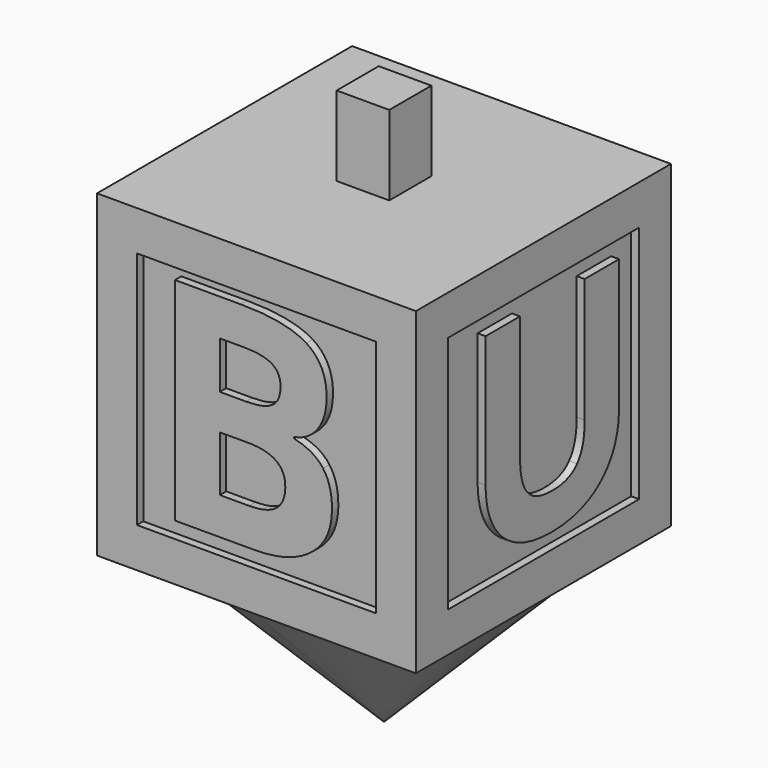
from build123d import *

# Parameters (mm, degrees)
F0_W      = 50.8
F0_H      = 50.8
F1_DEPTH  = 50.8
F2_W      = 38.1
F2_H      = 38.1
F3_DEPTH  = 1.27
F4_W      = 38.1
F4_H      = 38.1
F5_DEPTH  = 1.27
F6_W      = 38.1
F6_H      = 38.1
F7_DEPTH  = 1.27
F8_W      = 38.1
F8_H      = 38.1
F9_DEPTH  = 1.27
F10_W     = 8.382
F10_H     = 8.382
F11_DEPTH = 12.7
F13_DEPTH = 25.4
F14_SIZE  = 25.39999


# Not quite as in the source:
# - a fillet or chamfer is up to 0.001 mm smaller than in the source, because OpenCascade refuses the exact size


with BuildPart() as f1:
    # F0 (on Top) → F1 (new body)
    with BuildSketch(Plane.XY):
        Rectangle(F0_W, F0_H)
    extrude(amount=F1_DEPTH)

    # F2 (on face) → F3 (cut)
    with BuildSketch(Plane.XZ.offset(25.4)):
        with Locations((0, 25.4)):
            Rectangle(F2_W, F2_H)
        with BuildLine():
            Line((-12.9850329568, 8.9432131499), (-12.9850329568, 42.6816119349))
            Line((-12.9850329568, 42.6816119349), (-2.484703985, 42.6816119349))
            add(Edge.make_bspline(
                [(-2.484703985, 42.6816119349), (4.6927360717, 42.6816119349), (7.9343988133, 40.6398813015)],
                knots=[0, 0, 0, 1, 1, 1], degree=2))
            add(Edge.make_bspline(
                [(7.9343988133, 40.6398813015), (11.176061555, 38.5981506681), (11.176061555, 34.1454795218)],
                knots=[0, 0, 0, 1, 1, 1], degree=2))
            add(Edge.make_bspline(
                [(11.176061555, 34.1454795218), (11.176061555, 31.1179585102), (9.7582956179, 29.1796066431)],
                knots=[0, 0, 0, 1, 1, 1], degree=2))
            add(Edge.make_bspline(
                [(9.7582956179, 29.1796066431), (8.3405296807, 27.2412547759), (5.9849706498, 26.8498923037)],
                knots=[0, 0, 0, 1, 1, 1], degree=2))
            Line((5.9849706498, 26.8498923037), (5.9849706498, 26.6209821784))
            add(Edge.make_bspline(
                [(5.9849706498, 26.6209821784), (9.1897124035, 25.9047150123), (10.6111704394, 23.9442105523)],
                knots=[0, 0, 0, 1, 1, 1], degree=2))
            add(Edge.make_bspline(
                [(10.6111704394, 23.9442105523), (12.0326284753, 21.9837060924), (12.0326284753, 18.7272749556)],
                knots=[0, 0, 0, 1, 1, 1], degree=2))
            add(Edge.make_bspline(
                [(12.0326284753, 18.7272749556), (12.0326284753, 14.1121514623), (8.694971165, 11.5276823061)],
                knots=[0, 0, 0, 1, 1, 1], degree=2))
            add(Edge.make_bspline(
                [(8.694971165, 11.5276823061), (5.3573138547, 8.9432131499), (-0.3654392769, 8.9432131499)],
                knots=[0, 0, 0, 1, 1, 1], degree=2))
            Line((-0.3654392769, 8.9432131499), (-12.9850329568, 8.9432131499))
        make_face(mode=Mode.SUBTRACT)
        with BuildLine():
            Line((-5.8297454929, 36.8185590491), (-5.8297454929, 29.3162142985))
            Line((-5.8297454929, 29.3162142985), (-1.6798264478, 29.3162142985))
            add(Edge.make_bspline(
                [(-1.6798264478, 29.3162142985), (1.2295474023, 29.3162142985), (2.5328582768, 30.2170864044)],
                knots=[0, 0, 0, 1, 1, 1], degree=2))
            add(Edge.make_bspline(
                [(2.5328582768, 30.2170864044), (3.8361691513, 31.1179585102), (3.8361691513, 33.1929180328)],
                knots=[0, 0, 0, 1, 1, 1], degree=2))
            add(Edge.make_bspline(
                [(3.8361691513, 33.1929180328), (3.8361691513, 35.1349619988), (2.4184032142, 35.9767605239)],
                knots=[0, 0, 0, 1, 1, 1], degree=2))
            add(Edge.make_bspline(
                [(2.4184032142, 35.9767605239), (1.0006372771, 36.8185590491), (-2.07118892, 36.8185590491)],
                knots=[0, 0, 0, 1, 1, 1], degree=2))
            Line((-2.07118892, 36.8185590491), (-5.8297454929, 36.8185590491))
        make_face()
        with BuildLine():
            Line((-1.3992269394, 23.64515055), (-5.8297454929, 23.64515055))
            Line((-5.8297454929, 23.64515055), (-5.8297454929, 14.8505712213))
            Line((-5.8297454929, 14.8505712213), (-1.1703168141, 14.8505712213))
            add(Edge.make_bspline(
                [(-1.1703168141, 14.8505712213), (1.7833622215, 14.8505712213), (3.1900518623, 15.9803534524)],
                knots=[0, 0, 0, 1, 1, 1], degree=2))
            add(Edge.make_bspline(
                [(3.1900518623, 15.9803534524), (4.596741503, 17.1101356836), (4.596741503, 19.4435421217)],
                knots=[0, 0, 0, 1, 1, 1], degree=2))
            add(Edge.make_bspline(
                [(4.596741503, 19.4435421217), (4.596741503, 23.64515055), (-1.3992269394, 23.64515055)],
                knots=[0, 0, 0, 1, 1, 1], degree=2))
        make_face()
    extrude(amount=-F3_DEPTH, mode=Mode.SUBTRACT)

    # F4 (on face) → F5 (cut)
    with BuildSketch(Plane.YZ.offset(25.4)):
        with Locations((0, 25.4)):
            Rectangle(F4_W, F4_H)
        with BuildLine():
            Line((8.2110515278, 41.6381866004), (15.0563287647, 41.6381866004))
            Line((15.0563287647, 41.6381866004), (15.0563287647, 20.6913548071))
            add(Edge.make_bspline(
                [(15.0563287647, 20.6913548071), (15.0563287647, 17.098647189), (13.4513025803, 14.3988018192)],
                knots=[0, 0, 0, 1, 1, 1], degree=2))
            add(Edge.make_bspline(
                [(13.4513025803, 14.3988018192), (11.8462763959, 11.6989564493), (8.8098361308, 10.2569130563)],
                knots=[0, 0, 0, 1, 1, 1], degree=2))
            add(Edge.make_bspline(
                [(8.8098361308, 10.2569130563), (5.7733958658, 8.8148696632), (1.6350502071, 8.8148696632)],
                knots=[0, 0, 0, 1, 1, 1], degree=2))
            add(Edge.make_bspline(
                [(1.6350502071, 8.8148696632), (-4.6078993227, 8.8148696632), (-8.0624258786, 12.0178358237)],
                knots=[0, 0, 0, 1, 1, 1], degree=2))
            add(Edge.make_bspline(
                [(-8.0624258786, 12.0178358237), (-11.5169524345, 15.2208019843), (-11.5169524345, 20.776389307)],
                knots=[0, 0, 0, 1, 1, 1], degree=2))
            Line((-11.5169524345, 20.776389307), (-11.5169524345, 41.6381866004))
            Line((-11.5169524345, 41.6381866004), (-4.6787614059, 41.6381866004))
            Line((-4.6787614059, 41.6381866004), (-4.6787614059, 21.81806193))
            add(Edge.make_bspline(
                [(-4.6787614059, 21.81806193), (-4.6787614059, 18.0765439371), (-3.1729421379, 16.3262504822)],
                knots=[0, 0, 0, 1, 1, 1], degree=2))
            add(Edge.make_bspline(
                [(-3.1729421379, 16.3262504822), (-1.66712287, 14.5759570272), (1.8122054151, 14.5759570272)],
                knots=[0, 0, 0, 1, 1, 1], degree=2))
            add(Edge.make_bspline(
                [(1.8122054151, 14.5759570272), (5.178154367, 14.5759570272), (6.6946029474, 16.3368797946)],
                knots=[0, 0, 0, 1, 1, 1], degree=2))
            add(Edge.make_bspline(
                [(6.6946029474, 16.3368797946), (8.2110515278, 18.0978025621), (8.2110515278, 21.8605791799)],
                knots=[0, 0, 0, 1, 1, 1], degree=2))
            Line((8.2110515278, 21.8605791799), (8.2110515278, 41.6381866004))
        make_face(mode=Mode.SUBTRACT)
    extrude(amount=-F5_DEPTH, mode=Mode.SUBTRACT)

    # F6 (on face) → F7 (cut)
    with BuildSketch(Plane(origin=(0, 25.4, 0), x_dir=(-1, 0, 0), z_dir=(0, 1, 0))):
        with Locations((0, 25.4)):
            Rectangle(F6_W, F6_H)
        Polygon((-0.3206622132, 36.6013397979), (-0.3206622132, 8.6884368211), (-7.5084387172, 8.6884368211), (-7.5084387172, 36.6013397979), (-16.713836696, 36.6013397979), (-16.713836696, 42.5800269622), (8.8773180396, 42.5800269622), (8.8773180396, 36.6013397979), align=None, mode=Mode.SUBTRACT)
    extrude(amount=-F7_DEPTH, mode=Mode.SUBTRACT)

    # F8 (on face) → F9 (cut)
    with BuildSketch(Plane(origin=(-25.4, 0, 0), x_dir=(0, -1, 0), z_dir=(-1, 0, 0))):
        with Locations((0, 25.4)):
            Rectangle(F8_W, F8_H)
        Polygon((0.4234320166, 35.945847888), (0.4234320166, 10.2160740644), (-6.2021727762, 10.2160740644), (-6.2021727762, 35.945847888), (-14.6875964581, 35.945847888), (-14.6875964581, 41.4569288611), (8.902018129, 41.4569288611), (8.902018129, 35.945847888), align=None, mode=Mode.SUBTRACT)
    extrude(amount=-F9_DEPTH, mode=Mode.SUBTRACT)

    # F10 (on face) → F11 (join)
    with BuildSketch(Plane.XY.offset(50.8)):
        Rectangle(F10_W, F10_H)
    extrude(amount=F11_DEPTH)

    # F12 (on face) → F13 (join)
    with BuildSketch(Plane(origin=(0, 0, 0), x_dir=(1, 0, 0), z_dir=(0, 0, -1))):
        with BuildLine():
            ThreePointArc((3.01e-08, -25.4), (17.9605122528, -17.9605122315), (25.4, 0))
            ThreePointArc((25.4, 0), (17.9605122594, 17.9605122249), (4.89e-08, 25.4))
            ThreePointArc((4.89e-08, 25.4), (-17.9605122127, 17.9605122716), (-25.4, 3.44e-08))
            ThreePointArc((-25.4, 3.44e-08), (-17.9605122437, -17.9605122406), (3.01e-08, -25.4))
        make_face()
    extrude(amount=F13_DEPTH)

    # F14 (size 25.4 in the source; OpenCascade refuses exactly that, so slightly less here)
    f14_edges = [f1.edges().sort_by_distance(p)[0] for p in [
        (0, -25.4, -25.4),
    ]]
    chamfer(f14_edges, length=F14_SIZE)


solid = f1.part
